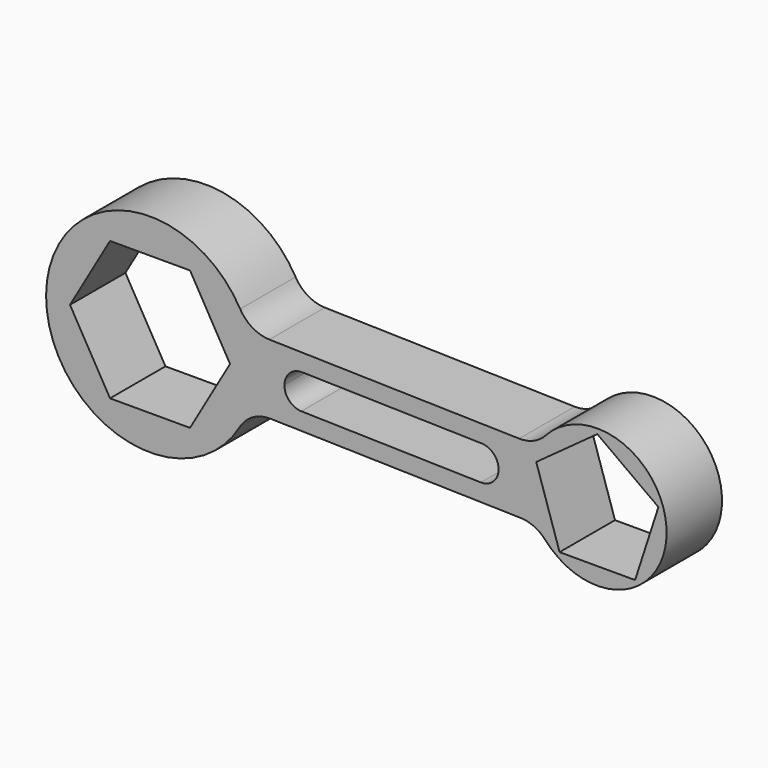
from build123d import *

# Parameters (mm, degrees)
F1_DEPTH = 508


# Not quite as in the source:
# - a feature names something its author has since deleted; it is built from what else it names


with BuildPart() as f1:
    # F0 (on Front) → F1 (new body)
    with BuildSketch(Plane.XZ):
        with BuildLine():
            ThreePointArc((90.8717905063, -26.9446916266), (60.5867734993, 146.7906129627), (-8.8258541664, 308.9110170961))
            ThreePointArc((-8.8258541664, 308.9110170961), (-1431.9038743199, -67.6123663617), (-11.2682681042, -453.2487029361))
            ThreePointArc((-11.2682681042, -453.2487029361), (65.7984429314, -268.4990677015), (92.0922130555, -70.0542559229))
            ThreePointArc((92.0922130555, -70.0542559229), (91.7870463114, -48.4908380293), (90.8717905063, -26.9446916266))
        make_face()
        Polygon((-83.3199134478, -70.0542559229), (-376.6138501962, -578.0542559229), (-963.2017236928, -578.0542559229), (-1256.4956604412, -70.0542559229), (-963.2017236928, 437.9457440771), (-376.6138501962, 437.9457440771), align=None, mode=Mode.SUBTRACT)
        with BuildLine():
            ThreePointArc((2230.3710697662, -455.9083929118), (2790.4957209899, -592.8162662797), (3117.7431527799, -118.0610566342))
            ThreePointArc((3117.7431527799, -118.0610566342), (2791.6202241037, 356.2644971015), (2231.9764955882, 221.5804495369))
            ThreePointArc((2231.9764955882, 221.5804495369), (2101.7445790707, -116.8572670267), (2230.3710697662, -455.9083929118))
        make_face()
        Polygon((2609.7431527799, 352.8808427932), (3057.6355150268, 27.4679936521), (2886.5558559499, -499.0610566342), (2332.9304496099, -499.0610566342), (2161.850790533, 27.4679936521), align=None, mode=Mode.SUBTRACT)
        with BuildLine():
            ThreePointArc((2230.3710697662, -455.9083929118), (2101.7445790707, -116.8572670267), (2231.9764955882, 221.5804495369))
            ThreePointArc((2231.9764955882, 221.5804495369), (2143.7064538419, 158.1782052373), (2037.0163567757, 137.4739051975))
            Line((2037.0163567757, 137.4739051975), (205.4579798763, 181.3054773441))
            ThreePointArc((205.4579798763, 181.3054773441), (81.5760518671, 216.9972910394), (-8.8258541664, 308.9110170961))
            ThreePointArc((-8.8258541664, 308.9110170961), (60.5867734993, 146.7906129627), (90.8717905063, -26.9446916266))
            ThreePointArc((90.8717905063, -26.9446916266), (91.7870463114, -48.4908380293), (92.0922130555, -70.0542559229))
            ThreePointArc((92.0922130555, -70.0542559229), (65.7984429314, -268.4990677015), (-11.2682681042, -453.2487029361))
            ThreePointArc((-11.2682681042, -453.2487029361), (84.287618689, -359.2994998742), (214.3550483926, -327.0528878488))
            Line((214.3550483925, -327.0528878488), (2046.761838476, -370.9047636255))
            ThreePointArc((2046.761838476, -370.9047636255), (2147.3957483239, -394.3351582008), (2230.3710697662, -455.9083929118))
        make_face()
        with BuildLine():
            ThreePointArc((439.4645539871, -205.4036891617), (350.5776252706, -166.0684205619), (315.5393103829, -75.4016353409))
            ThreePointArc((315.5393103829, -75.4016353409), (354.8745789827, 13.4852933757), (445.5413642038, 48.5236082633))
            Line((445.5413642038, 48.5236082633), (1761.7314269061, 17.0254696183))
            ThreePointArc((1761.7314269061, 17.0254696183), (1850.6183556226, -22.3097989815), (1885.6566705103, -112.9765842025))
            ThreePointArc((1885.6566705103, -112.9765842025), (1846.3214019105, -201.8635129191), (1755.6546166894, -236.9018278067))
            Line((1755.6546166894, -236.9018278067), (439.4645539871, -205.4036891617))
        make_face(mode=Mode.SUBTRACT)
    extrude(amount=F1_DEPTH)


solid = f1.part
